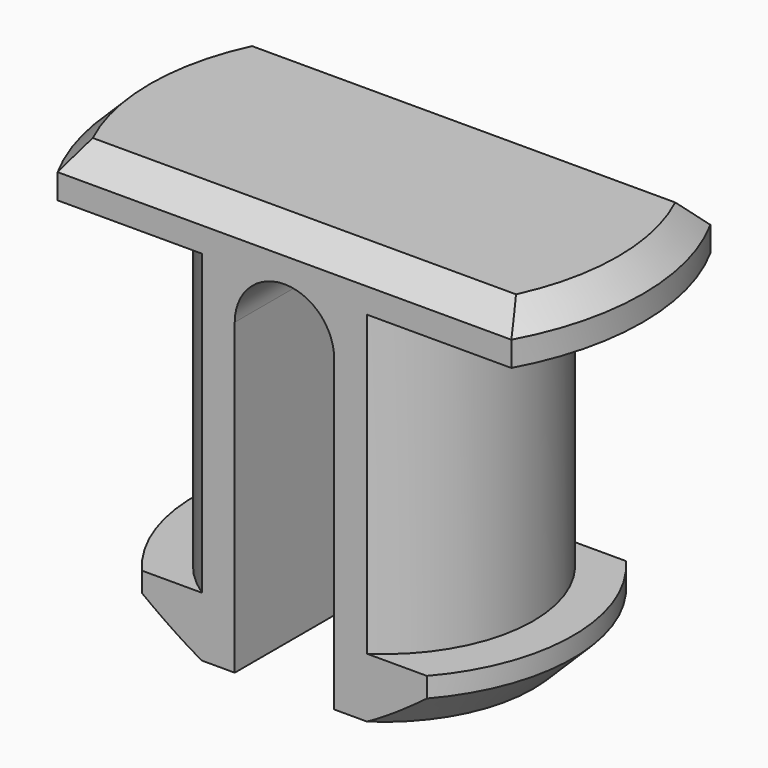
from build123d import *

# Parameters (mm, degrees)
F2_W          = 32.7764776534
F2_H          = 9.1045777517
F2_W_2        = 20.9091340361
F2_H_2        = 3.5162510286
F3_DEPTH      = 25
F4_W          = 2
F4_H          = 7.2
F5_DEPTH      = 25
F5_DEPTH_BACK = 25
F6_R          = 0.99999
F7_SIZE       = 0.8
F8_SIZE       = 0.5


# Not quite as in the source:
# - a fillet or chamfer is up to 0.001 mm smaller than in the source, because OpenCascade refuses the exact size


with BuildPart() as f1:
    # F0 (on Front) → F1 (revolve)
    with BuildSketch(Plane.XZ):
        Polygon((0, 0), (0, 8.2), (-5.2, 8.2), (-5.2, 7.2), (-3, 7.2), (-3, 1.2), (-3.8, 1.2), (-3.8, 0), align=None)
    revolve(axis=Axis((0, 0, 4.1), (0, 0, 1)))

    # F2 (on Top) → F3 (cut)
    with BuildSketch(Plane.XY):
        with Locations((1.9882628694, 7.0522888758)):
            Rectangle(F2_W, F2_H)
        with Locations((1.9568684145, -4.2581255143)):
            Rectangle(F2_W_2, F2_H_2)
    extrude(amount=F3_DEPTH, mode=Mode.SUBTRACT)

    # F4 (on Front) → F5 (cut, two sides)
    with BuildSketch(Plane.XZ) as f5_sk:
        with Locations((0, 3.6)):
            Rectangle(F4_W, F4_H)
    extrude(amount=-F5_DEPTH, mode=Mode.SUBTRACT)
    extrude(f5_sk.sketch, amount=F5_DEPTH_BACK, mode=Mode.SUBTRACT)

    # F6 (radius 1 in the source; OpenCascade refuses exactly that, so slightly less here)
    f6_edges = [f1.edges().sort_by_distance(p)[0] for p in [
        (-1, 0, 7.2),
        (1, 0, 7.2),
    ]]
    fillet(f6_edges, radius=F6_R)

    # F7
    f7_edges = [f1.edges().sort_by_distance(p)[0] for p in [
        (3.8, 0, 0),
        (-3.8, 0, 0),
    ]]
    chamfer(f7_edges, length=F7_SIZE)

    # F8
    f8_edges = [f1.edges().sort_by_distance(p)[0] for p in [
        (0, -2.5, 8.2),
        (-5.2, 0, 8.2),
        (0, 2.5, 8.2),
        (5.2, 0, 8.2),
    ]]
    chamfer(f8_edges, length=F8_SIZE)


solid = f1.part
